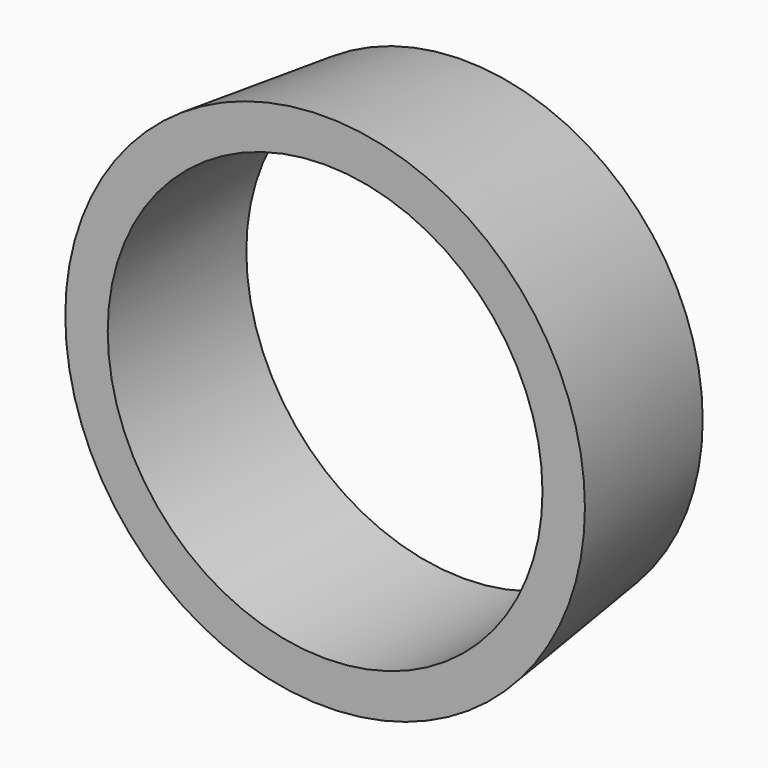
from build123d import *

# Parameters (mm, degrees)
F0_R     = 37.5
F0_R_2   = 31.375
F1_DEPTH = 25
F2_SIZE2 = 2.99999
F2_SIZE  = 24.99999


# Not quite as in the source:
# - a fillet or chamfer is up to 0.001 mm smaller than in the source, because OpenCascade refuses the exact size


with BuildPart() as f1:
    # F0 (on Front) → F1 (new body)
    with BuildSketch(Plane.XZ):
        Circle(F0_R)
        Circle(F0_R_2, mode=Mode.SUBTRACT)
    extrude(amount=F1_DEPTH)

    # F2 (size 25 and 3 in the source; OpenCascade refuses exactly that, so slightly less here)
    f2_edges = [f1.edges().sort_by_distance(p)[0] for p in [
        (-37.5, 0, 0),
    ]]
    f2_side = f1.faces().sort_by_distance((-37.5, -12.5, 0))[0]
    chamfer(f2_edges, length=F2_SIZE, length2=F2_SIZE2, reference=f2_side)


solid = f1.part
